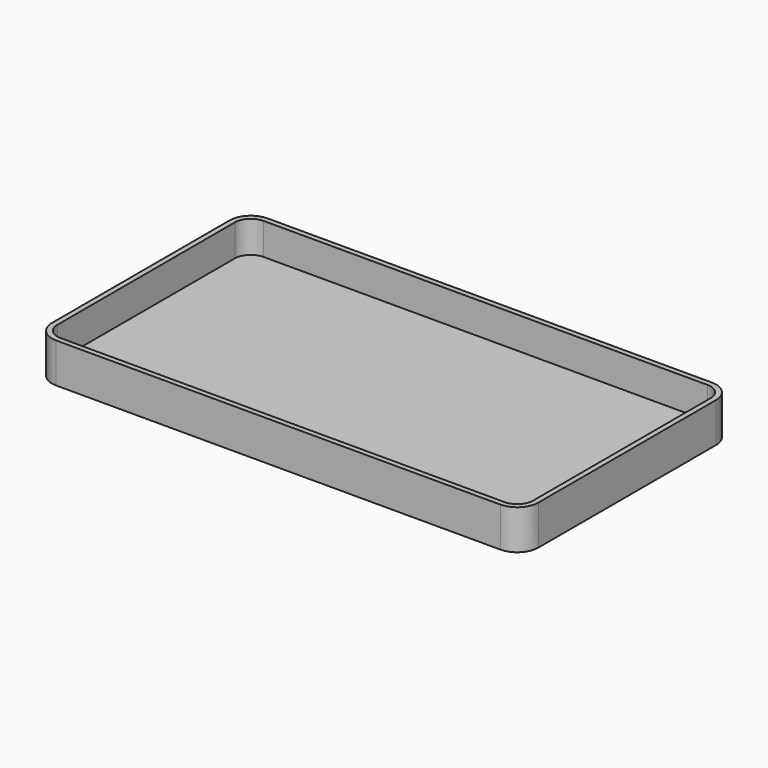
from build123d import *

# Parameters (mm, degrees)
F1_DEPTH = 19.05
F3_DEPTH = 76.2


# Not quite as in the source:
# - a feature names something its author has since deleted; it is built from what else it names


with BuildPart() as f1:
    # F0 (on Top) → F1 (new body)
    with BuildSketch(Plane.XY):
        with BuildLine():
            Line((533.4, 317.5), (-533.4, 317.5))
            ThreePointArc((-533.4, 317.5), (-569.3210244843, 302.6210244843), (-584.2, 266.7))
            Line((-584.2, 266.7), (-584.2, -266.7))
            ThreePointArc((-584.2, -266.7), (-569.3210244843, -302.6210244843), (-533.4, -317.5))
            Line((-533.4, -317.5), (533.4, -317.5))
            ThreePointArc((533.4, -317.5), (569.3210244843, -302.6210244843), (584.2, -266.7))
            Line((584.2, -266.7), (584.2, 266.7))
            ThreePointArc((584.2, 266.7), (569.3210244843, 302.6210244843), (533.4, 317.5))
        make_face()
    extrude(amount=F1_DEPTH)

    # F2 (on face) → F3 (join)
    with BuildSketch(Plane.XY.offset(19.05)):
        with BuildLine():
            ThreePointArc((584.2, 266.7), (569.3210244843, 302.6210244843), (533.4, 317.5))
            Line((533.4, 317.5), (-533.4, 317.5))
            ThreePointArc((-533.4, 317.5), (-569.3210244843, 302.6210244843), (-584.2, 266.7))
            Line((-584.2, 266.7), (-584.2, -266.7))
            ThreePointArc((-584.2, -266.7), (-569.3210244843, -302.6210244843), (-533.4, -317.5))
            Line((-533.4, -317.5), (533.4, -317.5))
            ThreePointArc((533.4, -317.5), (569.3210244843, -302.6210244843), (584.2, -266.7))
            Line((584.2, -266.7), (584.2, 266.7))
        make_face()
        with BuildLine():
            Line((-571.5, -266.7), (-571.5, 266.7))
            ThreePointArc((-571.5, 266.7), (-560.3407683632, 293.6407683632), (-533.4, 304.8))
            Line((-533.4, 304.8), (533.4, 304.8))
            ThreePointArc((533.4, 304.8), (560.3407683632, 293.6407683632), (571.5, 266.7))
            Line((571.5, 266.7), (571.5, -266.7))
            ThreePointArc((571.5, -266.7), (560.3407683632, -293.6407683632), (533.4, -304.8))
            Line((533.4, -304.8), (-533.4, -304.8))
            ThreePointArc((-533.4, -304.8), (-560.3407683632, -293.6407683632), (-571.5, -266.7))
        make_face(mode=Mode.SUBTRACT)
    extrude(amount=F3_DEPTH)


solid = f1.part
